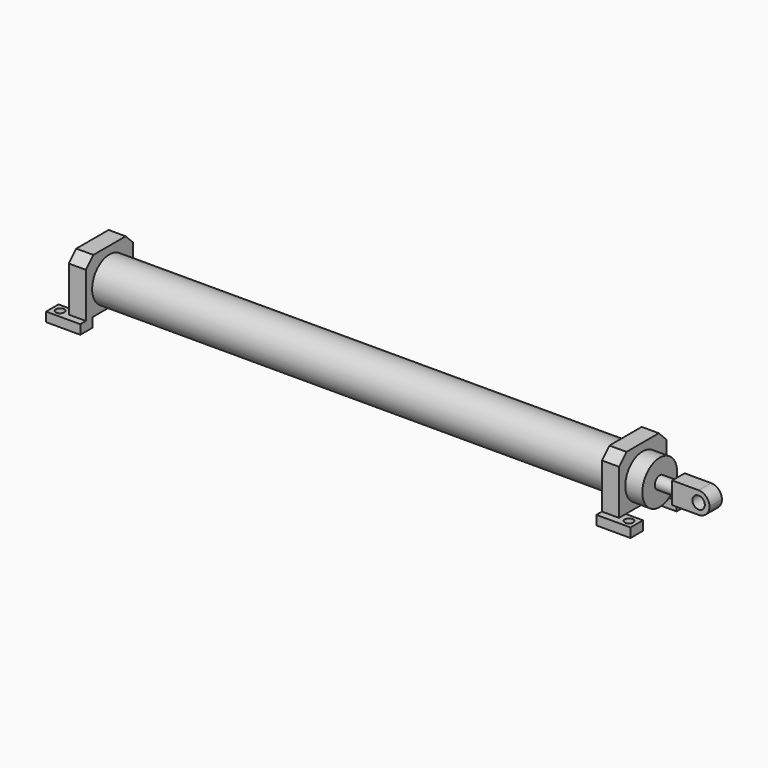
from build123d import *

# Parameters (mm, degrees)
F0_W      = 69.85
F0_H      = 31.75
F0_R      = 8.763
F1_DEPTH  = 19.05
F3_W      = 34.925
F3_H      = 120.65
F4_DEPTH  = 110.998
F5_SIZE   = 19.05
F8_R      = 44.45
F9_DEPTH  = 1123.95
F11_R     = 12.7
F12_DEPTH = 1016
F14_W     = 31.75
F14_H     = 44.45
F15_DEPTH = 76.2
F16_R     = 22.22499
F18_D     = 25.4


# Not quite as in the source:
# - a fillet or chamfer is up to 0.001 mm smaller than in the source, because OpenCascade refuses the exact size


with BuildPart() as f1:
    # F0 (on Top) → F1 (new body)
    with BuildSketch(Plane.XY):
        with Locations((-561.975, -58.801)):
            Rectangle(F0_W, F0_H)
        with Locations((-581.025, -58.674)):
            Circle(F0_R, mode=Mode.SUBTRACT)
    extrude(amount=F1_DEPTH)


with BuildPart() as f2_1:
    # F2: instance of F1
    add(f1.part.mirror(Plane.XZ))


with BuildPart() as f1_1:
    add(f1.part)

    add(f2_1.part)  # F4 merges F2_1
    # F3 (on face) → F4 (join)
    with BuildSketch(Plane.XY.offset(19.05)):
        with Locations((-544.5125, 0)):
            Rectangle(F3_W, F3_H)
    extrude(amount=F4_DEPTH)

    # F5
    f5_edges = [f1_1.edges().sort_by_distance(p)[0] for p in [
        (-544.5125, 60.325, 130.048),
        (-544.5125, -60.325, 130.048),
    ]]
    chamfer(f5_edges, length=F5_SIZE)

    # F6: union 


with BuildPart() as f7_1:
    # F7: instance of F1
    add(f1_1.part.mirror(Plane.YZ))


with BuildPart() as f1_2:
    add(f1_1.part)

    add(f7_1.part)  # F9 merges F7_1
    # F8 (on face) → F9 (join, through all)
    with BuildSketch(Plane.YZ.offset(596.9)):
        with Locations((0, 69.85)):
            Circle(F8_R)
    extrude(amount=-F9_DEPTH)


with BuildPart() as f12:
    # F11 (on offset) → F12 (new body)
    with BuildSketch(Plane.YZ.offset(673.1)):
        with Locations((0, 69.85)):
            Circle(F11_R)
    extrude(amount=-F12_DEPTH)

    # F14 (on offset) → F15 (join)
    with BuildSketch(Plane.YZ.offset(635)):
        with Locations((0, 69.85)):
            Rectangle(F14_W, F14_H)
    extrude(amount=F15_DEPTH)

    # F16 (radius 22.225 in the source; OpenCascade refuses exactly that, so slightly less here)
    f16_edges = [f12.edges().sort_by_distance(p)[0] for p in [
        (711.2, 0, 92.075),
        (711.2, 0, 47.625),
    ]]
    fillet(f16_edges, radius=F16_R)

    # F18 (through all)
    with Locations(Plane.XZ.offset(15.875)):
        with Locations((688.975, 69.85)):
            Hole(F18_D / 2)


solid = Compound([f1_2.part, f12.part])
